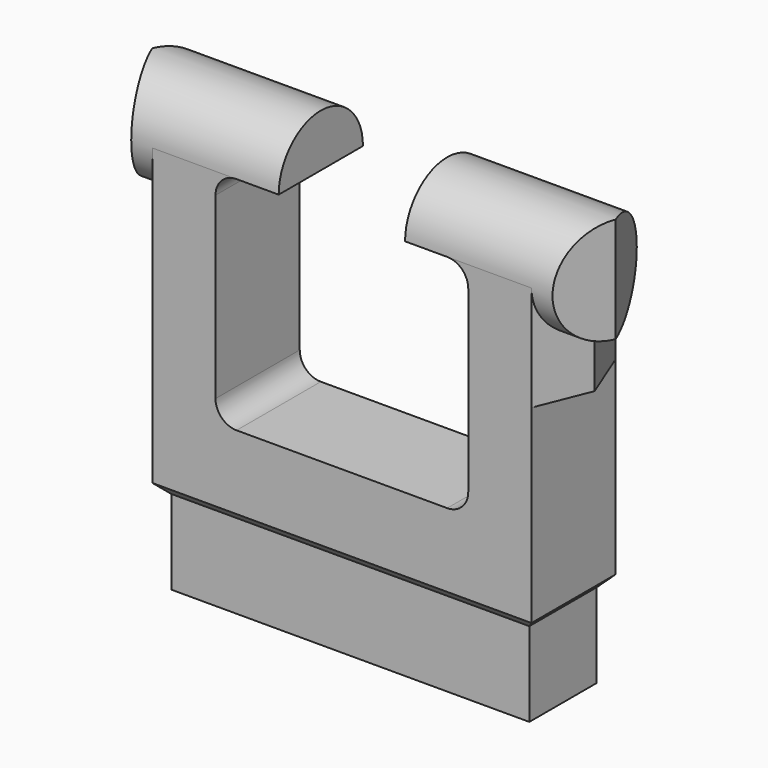
from build123d import *

# Parameters (mm, degrees)
F2_DEPTH    = 2.5
F3_DEPTH    = 10
F4_DEPTH    = 3
F5_DEPTH    = 6
F6_T1_DEPTH = 5
F8_DEPTH    = 14
F9_DEPTH    = 9
F10_DEPTH   = 1
F11_DEPTH   = 16.5
F12_FACE_W  = 18
F12_FACE_H  = 5
F13_DEPTH   = 0.5
F13_TAPER   = 45
F14_DEPTH   = 4


# Not quite as in the source:
# - a fillet or chamfer that OpenCascade refuses, or shapes differently, is made with other operations: its cross-section is extruded or revolved along the edge and cut away or added


with BuildPart() as f2:
    # F0 (on Front) → F2 (new body, symmetric)
    with BuildSketch(Plane.XZ):
        Polygon((0, 3.5), (0, 0), (9, 0), (9, 14), (6, 14), (6, 3.5), align=None)
    extrude(amount=F2_DEPTH, both=True)

    # F1 (on Right) → F3 (join)
    with BuildSketch(Plane.YZ):
        with BuildLine():
            Line((-2.5, 14), (2.5, 14))
            ThreePointArc((2.5, 14), (0, 16.5), (-2.5, 14))
        make_face()
        with BuildLine():
            ThreePointArc((-2.5, 14), (0, 11.5), (2.5, 14))
            Line((2.5, 14), (-2.5, 14))
        make_face()
    extrude(amount=F3_DEPTH)

    # F1 (on Right) → F4 (cut)
    with BuildSketch(Plane.YZ):
        with BuildLine():
            Line((-2.5, 14), (2.5, 14))
            ThreePointArc((2.5, 14), (0, 16.5), (-2.5, 14))
        make_face()
        with BuildLine():
            ThreePointArc((-2.5, 14), (0, 11.5), (2.5, 14))
            Line((2.5, 14), (-2.5, 14))
        make_face()
    extrude(amount=F4_DEPTH, mode=Mode.SUBTRACT)

    # F1 (on Right) → F5 (cut)
    with BuildSketch(Plane.YZ):
        with BuildLine():
            ThreePointArc((-2.5, 14), (0, 11.5), (2.5, 14))
            Line((2.5, 14), (-2.5, 14))
        make_face()
    extrude(amount=F5_DEPTH, mode=Mode.SUBTRACT)

    # F6: fillet of radius 1 on 2 edges, made by hand

    # F6_s2 → F6_t1 (join)
    with BuildSketch(Plane.XZ.offset(-2.5)):
        with BuildLine():
            ThreePointArc((6, 13), (5.7071067812, 13.7071067812), (5, 14))
            Line((5, 14), (6, 14))
            Line((6, 14), (6, 13))
        make_face()
        with BuildLine():
            ThreePointArc((5, 3.5), (5.7071067812, 3.7928932188), (6, 4.5))
            Line((6, 4.5), (6, 3.5))
            Line((6, 3.5), (5, 3.5))
        make_face()
    extrude(amount=F6_T1_DEPTH)

    # F7 (on Top) → F8 (join)
    with BuildSketch(Plane.XY):
        Polygon((9, 2.5), (9, -2.5), (10, 0), align=None)
    extrude(amount=F8_DEPTH)

    # F7 (on Top) → F9 (cut)
    with BuildSketch(Plane.XY):
        Polygon((9, 2.5), (9, -2.5), (10, 0), align=None)
    extrude(amount=F9_DEPTH, mode=Mode.SUBTRACT)

    # F10 (add): a face of the model
    f10_faces = [f2.faces().sort_by_distance(p)[0] for p in [
        (10, -1.717766953, 12.282233047),
    ]]
    extrude(f10_faces, amount=F10_DEPTH)

    # F7 (on Top) → F11 (cut)
    with BuildSketch(Plane.XY):
        Polygon((11, 0), (10, -2.5), (11.5, -2.5), (11.5, 2.5), (10, 2.5), align=None)
    extrude(amount=F11_DEPTH, mode=Mode.SUBTRACT)

    # F12: F2 across face


with BuildPart() as f2_1:
    add(f2.part)
    add(f2.part.mirror(Plane(origin=(0, 0, 1.75), x_dir=(0, -1, 0), z_dir=(-1, 0, 0))))

    # F12_face (on face) → F13 (join)
    with BuildSketch(Plane(origin=(0, 0, 0), x_dir=(1, 0, 0), z_dir=(0, 0, -1))):
        Rectangle(F12_FACE_W, F12_FACE_H)
    extrude(amount=F13_DEPTH, taper=F13_TAPER)

    # F14 (add): a face of the model
    f14_faces = [f2_1.faces().sort_by_distance(p)[0] for p in [
        (0, 0, -0.5),
    ]]
    extrude(f14_faces, amount=F14_DEPTH)


solid = f2_1.part
